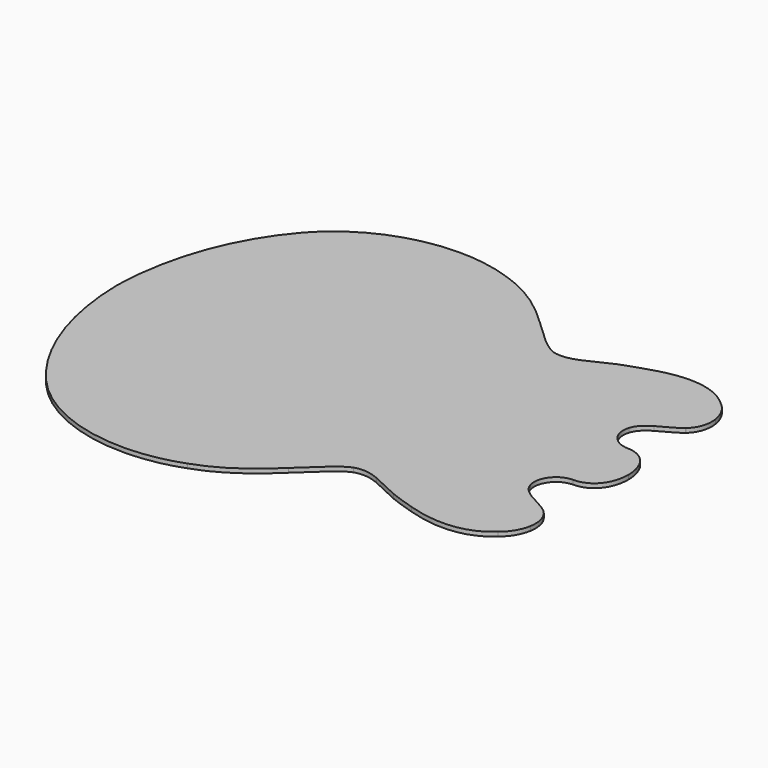
from build123d import *

# Parameters (mm, degrees)
F1_DEPTH = 4


# Not quite as in the source:
# - ends of sketch curves that miss each other by under 0.0002 mm in the source are joined


with BuildPart() as f1:
    # F0 (on Top) → F1 (new body)
    with BuildSketch(Plane.XY):
        with BuildLine():
            add(Edge.make_bspline(
                [(-23.29275, 188.71263), (-40.744167, 195.27633), (-59.410257, 198.41332), (-78.043821, 198.249744)],
                knots=[0, 0, 0, 0, 1, 1, 1, 1], degree=3))
            add(Edge.make_bspline(
                [(-78.043821, 198.249744), (-119.036105, 197.889891), (-160.001254, 181.57068), (-187.364696, 150.031637)],
                knots=[0, 0, 0, 0, 1, 1, 1, 1], degree=3))
            add(Edge.make_bspline(
                [(-187.364696, 150.031637), (-187.364865, 150.031442), (-187.364978, 150.031355), (-187.365261, 150.031072)],
                knots=[0, 0, 0, 0, 1, 1, 1, 1], degree=3))
            add(Edge.make_bspline(
                [(-187.365261, 150.031072), (-223.157197, 108.912672), (-239.83493, 53.349791), (-240.796196, -0.140351)],
                knots=[0, 0, 0, 0, 1, 1, 1, 1], degree=3))
            add(Edge.make_bspline(
                [(-240.796196, -0.140351), (-240.797267, -0.200062), (-240.797267, -0.259787), (-240.796196, -0.319498)],
                knots=[0, 0, 0, 0, 1, 1, 1, 1], degree=3))
            add(Edge.make_bspline(
                [(-240.796196, -0.319498), (-239.840937, -53.821863), (-222.970632, -108.900151), (-187.197127, -149.997041)],
                knots=[0, 0, 0, 0, 1, 1, 1, 1], degree=3))
            add(Edge.make_bspline(
                [(-187.197127, -149.997041), (-147.436926, -195.824596), (-79.112374, -209.648856), (-23.30153, -188.74031)],
                knots=[0, 0, 0, 0, 1, 1, 1, 1], degree=3))
            Line((-23.30153, -188.74031), (-23.130102, -188.679124))
            add(Edge.make_bspline(
                [(-23.130102, -188.679124), (1.059853, -180.570344), (21.278733, -165.037933), (38.938938, -147.973536)],
                knots=[0, 0, 0, 0, 1, 1, 1, 1], degree=3))
            add(Edge.make_bspline(
                [(38.938938, -147.973536), (52.026993, -136.892306), (62.204773, -123.641634), (75.896277, -117.517243)],
                knots=[0, 0, 0, 0, 1, 1, 1, 1], degree=3))
            add(Edge.make_bspline(
                [(75.896277, -117.517243), (83.85737, -115.06047), (91.397501, -116.61066), (99.542858, -119.902331)],
                knots=[0, 0, 0, 0, 1, 1, 1, 1], degree=3))
            add(Edge.make_bspline(
                [(99.542858, -119.902331), (107.756908, -123.2218), (116.195437, -128.328386), (125.148457, -131.870331)],
                knots=[0, 0, 0, 0, 1, 1, 1, 1], degree=3))
            add(Edge.make_bspline(
                [(125.148457, -131.870331), (132.727224, -134.996817), (140.627979, -137.381228), (148.394876, -139.826571)],
                knots=[0, 0, 0, 0, 1, 1, 1, 1], degree=3))
            add(Edge.make_bspline(
                [(148.394876, -139.826571), (148.394876, -139.826853), (148.397698, -139.826853), (148.397698, -139.826571)],
                knots=[0, 0, 0, 0, 1, 1, 1, 1], degree=3))
            add(Edge.make_bspline(
                [(148.397698, -139.826571), (148.40052, -139.826571), (148.401649, -139.829393), (148.403907, -139.829393)],
                knots=[0, 0, 0, 0, 1, 1, 1, 1], degree=3))
            add(Edge.make_bspline(
                [(148.403907, -139.829393), (172.528911, -147.473466), (202.043599, -149.701441), (222.443157, -131.039695)],
                knots=[0, 0, 0, 0, 1, 1, 1, 1], degree=3))
            Line((222.443157, -131.039695), (222.513713, -130.980174))
            add(Edge.make_bspline(
                [(222.513713, -130.980174), (229.464818, -125.631639), (234.197007, -117.510187), (235.635381, -108.839502)],
                knots=[0, 0, 0, 0, 1, 1, 1, 1], degree=3))
            add(Edge.make_bspline(
                [(235.635381, -108.839502), (237.078806, -100.138393), (234.900785, -90.513402), (227.492818, -83.846297)],
                knots=[0, 0, 0, 0, 1, 1, 1, 1], degree=3))
            add(Edge.make_bspline(
                [(227.492818, -83.846297), (227.400465, -83.76321), (227.305045, -83.683596), (227.206758, -83.607622)],
                knots=[0, 0, 0, 0, 1, 1, 1, 1], degree=3))
            add(Edge.make_bspline(
                [(227.206758, -83.607622), (220.687876, -78.567613), (213.176701, -75.418408), (207.090691, -71.705791)],
                knots=[0, 0, 0, 0, 1, 1, 1, 1], degree=3))
            add(Edge.make_bspline(
                [(207.090691, -71.705791), (201.005472, -67.993635), (196.586267, -64.15215), (194.627165, -57.863121)],
                knots=[0, 0, 0, 0, 1, 1, 1, 1], degree=3))
            add(Edge.make_bspline(
                [(194.627165, -57.863121), (194.626911, -57.862275), (194.627165, -57.86171), (194.627165, -57.860864)],
                knots=[0, 0, 0, 0, 1, 1, 1, 1], degree=3))
            add(Edge.make_bspline(
                [(194.627165, -57.860864), (190.811493, -45.539507), (200.792423, -32.097127), (214.099398, -32.108636)],
                knots=[0, 0, 0, 0, 1, 1, 1, 1], degree=3))
            add(Edge.make_bspline(
                [(214.099398, -32.108636), (214.100339, -32.108637), (214.10128, -32.108637), (214.10222, -32.108636)],
                knots=[0, 0, 0, 0, 1, 1, 1, 1], degree=3))
            add(Edge.make_bspline(
                [(214.10222, -32.108636), (222.998711, -32.113688), (230.233817, -27.742198), (234.609616, -21.595858)],
                knots=[0, 0, 0, 0, 1, 1, 1, 1], degree=3))
            add(Edge.make_bspline(
                [(234.609616, -21.595858), (238.985415, -15.449518), (240.879719, -7.737472), (240.796999, -0.090745)],
                knots=[0, 0, 0, 0, 1, 1, 1, 1], degree=3))
            add(Edge.make_bspline(
                [(240.796999, -0.090745), (240.714308, 7.555981), (238.653296, 15.239885), (234.273376, 21.375232)],
                knots=[0, 0, 0, 0, 1, 1, 1, 1], degree=3))
            add(Edge.make_bspline(
                [(234.273376, 21.375232), (229.893457, 27.51058), (222.80982, 31.975787), (214.131967, 32.074872)],
                knots=[0, 0, 0, 0, 1, 1, 1, 1], degree=3))
            add(Edge.make_bspline(
                [(214.131967, 32.074872), (200.3598011228, 32.409862366), (190.6341888263, 45.5397705426), (194.460767, 57.895973)],
                knots=[0.0012785739, 0.0012785739, 0.0012785739, 0.0012785739, 1, 1, 1, 1], degree=3))
            add(Edge.make_bspline(
                [(194.460767, 57.895973), (194.460993, 57.89682), (194.460767, 57.897384), (194.460767, 57.898231)],
                knots=[0, 0, 0, 0, 1, 1, 1, 1], degree=3))
            add(Edge.make_bspline(
                [(194.460767, 57.898231), (196.419841, 64.18724), (200.839074, 68.028874), (206.924293, 71.740898)],
                knots=[0, 0, 0, 0, 1, 1, 1, 1], degree=3))
            add(Edge.make_bspline(
                [(206.924293, 71.740898), (213.010274, 75.453396), (220.521421, 78.602146), (227.040331, 83.642189)],
                knots=[0, 0, 0, 0, 1, 1, 1, 1], degree=3))
            add(Edge.make_bspline(
                [(227.040331, 83.642189), (227.138629, 83.718163), (227.234058, 83.797777), (227.32642, 83.880865)],
                knots=[0, 0, 0, 0, 1, 1, 1, 1], degree=3))
            add(Edge.make_bspline(
                [(227.32642, 83.880865), (234.734386, 90.548), (236.91238, 100.173387), (235.468954, 108.87462)],
                knots=[0, 0, 0, 0, 1, 1, 1, 1], degree=3))
            add(Edge.make_bspline(
                [(235.468954, 108.87462), (234.0392708475, 117.493181786), (229.358044954, 125.5721274646), (222.4753975178, 130.9216294129)],
                knots=[0, 0, 0, 0, 0.9904989081, 0.9904989081, 0.9904989081, 0.9904989081], degree=3))
            add(Edge.make_bspline(
                [(222.4753975178, 130.9216294129), (202.2201967941, 149.6382929896), (173.4466709537, 148.1501016784), (149.669561, 140.174275)],
                knots=[0.0028310813, 0.0028310813, 0.0028310813, 0.0028310813, 1, 1, 1, 1], degree=3))
            add(Edge.make_bspline(
                [(149.669561, 140.174275), (147.849594, 139.64173), (141.739935, 137.657691), (138.376805, 136.671302)],
                knots=[0, 0, 0, 0, 1, 1, 1, 1], degree=3))
            add(Edge.make_bspline(
                [(138.376805, 136.671302), (138.337334, 136.659662), (138.298008, 136.647535), (138.258836, 136.634923)],
                knots=[0, 0, 0, 0, 1, 1, 1, 1], degree=3))
            add(Edge.make_bspline(
                [(138.258836, 136.634923), (130.579485, 134.174462), (132.826877, 134.841689), (125.095823, 131.950695)],
                knots=[0, 0, 0, 0, 1, 1, 1, 1], degree=3))
            add(Edge.make_bspline(
                [(125.095823, 131.950695), (125.066878, 131.939938), (125.038034, 131.928913), (125.009293, 131.917621)],
                knots=[0, 0, 0, 0, 1, 1, 1, 1], degree=3))
            add(Edge.make_bspline(
                [(125.009293, 131.917621), (116.046028, 128.375264), (107.599145, 123.260353), (99.376657, 119.937508)],
                knots=[0, 0, 0, 0, 1, 1, 1, 1], degree=3))
            add(Edge.make_bspline(
                [(99.376657, 119.937508), (91.231301, 116.645826), (83.69117, 115.095644), (75.730076, 117.5524)],
                knots=[0, 0, 0, 0, 1, 1, 1, 1], degree=3))
            add(Edge.make_bspline(
                [(75.730076, 117.5524), (62.038375, 123.676899), (51.860539, 136.927923), (38.772201, 148.009249)],
                knots=[0, 0, 0, 0, 1, 1, 1, 1], degree=3))
            add(Edge.make_bspline(
                [(38.772201, 148.009249), (21.11234, 165.071874), (0.895704, 180.602741), (-23.291056, 188.712066)],
                knots=[0, 0, 0, 0, 1, 1, 1, 1], degree=3))
            Line((-23.291056, 188.712066), (-23.29275, 188.71263))
        make_face()
        with BuildLine():
            add(Edge.make_bspline(
                [(222.4753975178, 130.9216294129), (222.4093775909, 130.9729430579), (222.3431551094, 131.0240055645), (222.276731, 131.074815)],
                knots=[0.9904989081, 0.9904989081, 0.9904989081, 0.9904989081, 1, 1, 1, 1], degree=3))
            add(Edge.make_bspline(
                [(222.647712, 130.761724), (222.5903427082, 130.8151888768), (222.5329044444, 130.8684905764), (222.4753975178, 130.9216294129)],
                knots=[0, 0, 0, 0, 0.0028310813, 0.0028310813, 0.0028310813, 0.0028310813], degree=3))
            Line((222.647712, 130.761724), (222.276731, 131.074815))
        make_face(mode=Mode.SUBTRACT)
        with BuildLine():
            add(Edge.make_bspline(
                [(222.647712, 130.761724), (222.5903427082, 130.8151888768), (222.5329044444, 130.8684905764), (222.4753975178, 130.9216294129)],
                knots=[0, 0, 0, 0, 0.0028310813, 0.0028310813, 0.0028310813, 0.0028310813], degree=3))
            add(Edge.make_bspline(
                [(222.4753975178, 130.9216294129), (222.4093775909, 130.9729430579), (222.3431551094, 131.0240055645), (222.276731, 131.074815)],
                knots=[0.9904989081, 0.9904989081, 0.9904989081, 0.9904989081, 1, 1, 1, 1], degree=3))
            Line((222.276731, 131.074815), (222.647712, 130.761724))
        make_face()
    extrude(amount=F1_DEPTH)


solid = f1.part
